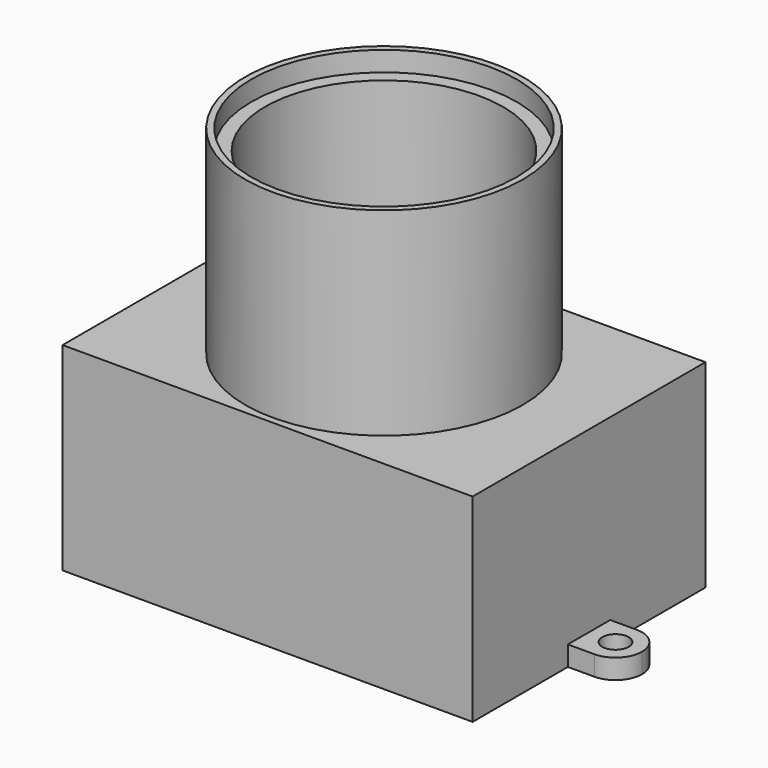
from build123d import *

# Parameters (mm, degrees)
F0_W          = 62
F0_H          = 44
F1_DEPTH      = 30
F1_DEPTH_BACK = 30
F2_W          = 62
F2_H          = 44
F2_R          = 21
F2_R_2        = 18
F3_DEPTH      = 30
F4_T          = 5
F5_R          = 2
F6_DEPTH      = 3
F7_R          = 9.05
F8_DEPTH      = 1.5
F9_R          = 18
F10_DEPTH     = 30.001
F11_R         = 20.05
F12_DEPTH     = 3


# Not quite as in the source:
# - a shell that OpenCascade refuses in one call is made with other operations: the cavity is built on its own and cut out


with BuildPart() as f1:
    # F0 (on Top) → F1 (new body, two sides)
    with BuildSketch(Plane.XY) as f1_sk:
        Rectangle(F0_W, F0_H)
    extrude(amount=F1_DEPTH)
    extrude(f1_sk.sketch, amount=-F1_DEPTH_BACK)

    # F2 (on face) → F3 (cut)
    with BuildSketch(Plane.XY.offset(30)):
        Rectangle(F2_W, F2_H)
        Circle(F2_R, mode=Mode.SUBTRACT)
        Circle(F2_R_2)
    extrude(amount=-F3_DEPTH, mode=Mode.SUBTRACT)

    # F4: shell of thickness 5, made by hand


with BuildPart() as f4_core1:
    # F4_t2: copy of F1
    add(f1.part)

    # the walls: a layer under each face that stays
    f4_faces = [f4_core1.faces().sort_by_distance(p)[0] for p in [
        (0, 22, -15),
        (31, 0, -15),
        (-31, 0, -15),
        (-20.6666666667, -14.6666666667, 0),
        (0, -22, -15),
        (-21, 0, 15),
        (-14, -14, 30),
        (-18, 0, 15),
        (0, 0, 0),
    ]]
    thicken(f4_faces, amount=-F4_T, mode=Mode.SUBTRACT)

    # F4_s3 → F4_t4 (revolve, cut)
    with BuildSketch(Plane.XZ):
        Polygon((21.05, 0.05), (21, -5), (16, -5), (16, 0), align=None)
    revolve(axis=Axis((0, 0, 0), (0, 0, 1)), mode=Mode.SUBTRACT)

    # F4_s5 → F4_t6 (revolve, cut)
    with BuildSketch(Plane.XZ):
        Polygon((17.95, 0.05), (23, 0), (23, -5), (18, -5), align=None)
    revolve(axis=Axis((0, 0, 0), (0, 0, 1)), mode=Mode.SUBTRACT)


with BuildPart() as f1_1:
    add(f1.part)

    # what is left inside the walls is the cavity
    f4_cavity = [f4_core1.part.solids().sort_by_distance(p)[0] for p in [
        (0, -5.666667, -29.95),
    ]]
    add(f4_cavity, mode=Mode.SUBTRACT)

    # F5 (on face) → F6 (join)
    with BuildSketch(Plane(origin=(0, 0, -30), x_dir=(1, 0, 0), z_dir=(0, 0, -1))):
        with BuildLine():
            Line((35, 4), (31, 4))
            Line((31, 4), (31, -4))
            Line((31, -4), (35, -4))
            ThreePointArc((35, -4), (37.8284271247, -2.8284271247), (39, 0))
            ThreePointArc((39, 0), (37.8284271247, 2.8284271247), (35, 4))
        make_face()
        with Locations((35, 0)):
            Circle(F5_R, mode=Mode.SUBTRACT)
        with BuildLine():
            ThreePointArc((-39, 0), (-37.8284271247, -2.8284271247), (-35, -4))
            Line((-35, -4), (-31, -4))
            Line((-31, -4), (-31, 4))
            Line((-31, 4), (-35, 4))
            ThreePointArc((-35, 4), (-37.8284271247, 2.8284271247), (-39, 0))
        make_face()
        with Locations((-35, 0)):
            Circle(F5_R, mode=Mode.SUBTRACT)
    extrude(amount=-F6_DEPTH)

    # F7 (on face) → F8 (cut)
    with BuildSketch(Plane.XY.offset(30)):
        Circle(F7_R)
    extrude(amount=-F8_DEPTH, mode=Mode.SUBTRACT)

    # F9 (on face) → F10 (cut, through all)
    with BuildSketch(Plane.XY):
        Circle(F9_R)
    extrude(amount=-F10_DEPTH, mode=Mode.SUBTRACT)

    # F11 (on face) → F12 (cut)
    with BuildSketch(Plane.XY.offset(30)):
        Circle(F11_R)
    extrude(amount=-F12_DEPTH, mode=Mode.SUBTRACT)


solid = f1_1.part
